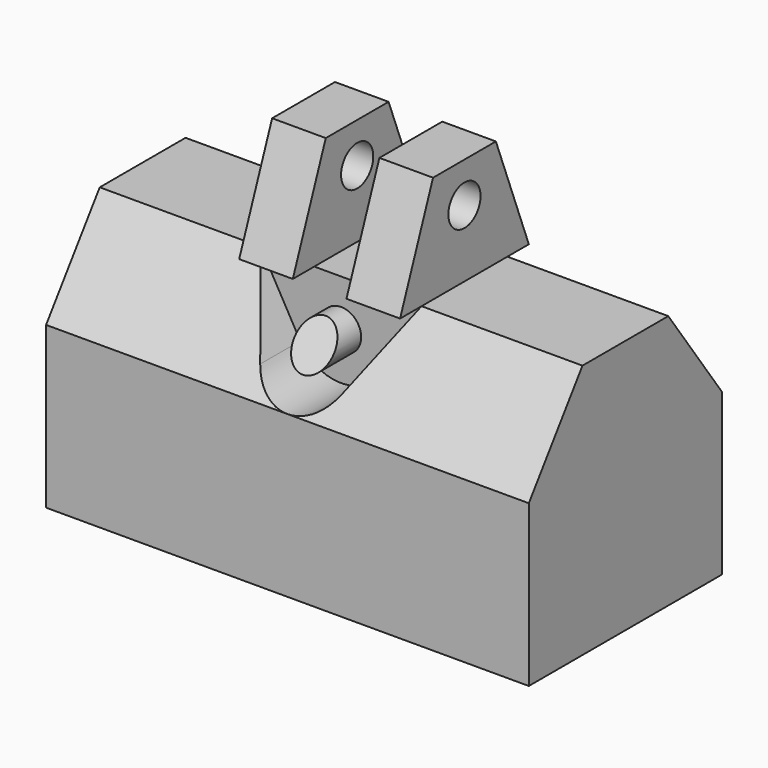
from build123d import *

# Parameters (mm, degrees)
F0_W      = 228.6
F0_H      = 114.3
F1_DEPTH  = 120.65
F6_R      = 9.525
F7_DEPTH  = 38.1
F8_DEPTH  = 12.7
F10_DEPTH = 228.6
F11_R     = 9.525
F12_DEPTH = 31.75


# Not quite as in the source:
# - a pattern or mirror of a feature is missing from the dataset's text; its kind, count and spacing are read off the source's solid


with BuildPart() as f1:
    # F0 (on Top) → F1 (new body)
    with BuildSketch(Plane.XY):
        with Locations((-114.3, 57.15)):
            Rectangle(F0_W, F0_H)
    extrude(amount=F1_DEPTH)

    # F6 (on 3pt) → F7 (join, symmetric)
    with BuildSketch(Plane(origin=(-114.3, 0, 0), x_dir=(0, -1, 0), z_dir=(-1, 0, 0))):
        Polygon((-75.7497070202, 171.45), (-95.25, 120.65), (-19.05, 120.65), (-38.5502929798, 171.45), align=None)
        with Locations((-57.15, 152.4)):
            Circle(F6_R, mode=Mode.SUBTRACT)
    extrude(amount=F7_DEPTH, both=True)

    # F6 (on 3pt) → F8 (cut, symmetric)
    with BuildSketch(Plane(origin=(-114.3, 0, 0), x_dir=(0, -1, 0), z_dir=(-1, 0, 0))):
        Polygon((-75.7497070202, 171.45), (-95.25, 120.65), (-19.05, 120.65), (-38.5502929798, 171.45), align=None)
        with Locations((-57.15, 152.4)):
            Circle(F6_R, mode=Mode.SUBTRACT)
    extrude(amount=F8_DEPTH, both=True, mode=Mode.SUBTRACT)

    # F9 (on face) → F10 (cut, through all)
    with BuildSketch(Plane.YZ):
        Polygon((31.75, 120.65), (0, 120.65), (0, 76.2), align=None)
        Polygon((114.3, 120.65), (82.55, 120.65), (114.3, 76.2), align=None)
    extrude(amount=-F10_DEPTH, mode=Mode.SUBTRACT)

    # F11 (on face) → F12 (cut)
    with BuildSketch(Plane.XZ):
        with BuildLine():
            Line((-152.4, 120.65), (-133.6461139863, 87.4852331607))
            ThreePointArc((-133.6461139892, 87.4852331591), (-114.3000000002, 76.2), (-94.9538860115, 87.4852331593))
            Line((-94.9538860135, 87.4852331605), (-76.2, 120.65))
            Line((-76.2, 120.65), (-152.4, 120.65))
        make_face()
        with Locations((-114.3000000004, 98.425)):
            Circle(F11_R, mode=Mode.SUBTRACT)
    f12 = extrude(amount=-F12_DEPTH, mode=Mode.SUBTRACT)

    # F12_copies: F12 across plane
    add(f12.mirror(Plane.ZX.offset(57.15)), mode=Mode.SUBTRACT)


solid = f1.part
